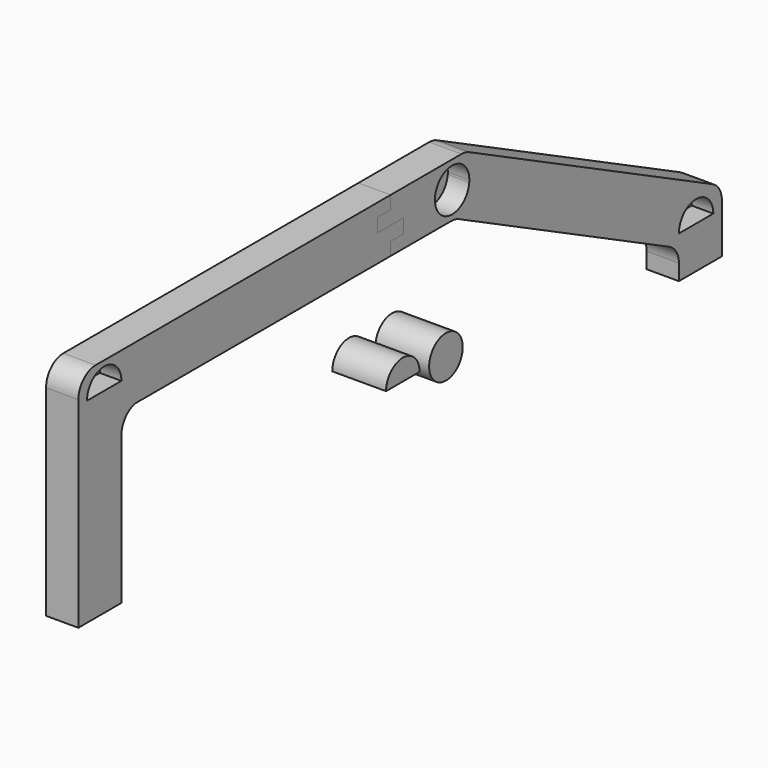
from build123d import *

# Parameters (mm, degrees)
F3_DEPTH  = 15
F4_DEPTH  = 25
F5_DEPTH  = 15
F6_DEPTH  = 25
F7_DEPTH  = 25
F8_R      = 9.75
F9_DEPTH  = 25
F10_DEPTH = 5
F11_DEPTH = 5
F12_DEPTH = 5


with BuildPart() as f3:
    # F2 (on Right) → F3 (new body)
    with BuildSketch(Plane.YZ):
        with BuildLine():
            Line((-64.0537443757, -47.7458898533), (-64.0537443757, -41.7458898533))
            Line((-64.0537443757, -41.7458898533), (-235.4606981414, -41.7458898533))
            ThreePointArc((-235.4606981414, -41.7458898533), (-242.5317659533, -44.6748220415), (-245.4606981414, -51.7458898533))
            Line((-245.4606981414, -51.7458898533), (-245.4606981414, -145.1103440631))
            Line((-245.4606981414, -145.1103440631), (-220.4606981414, -145.1103440631))
            Line((-220.4606981414, -145.1103440631), (-220.4606981414, -76.5684022923))
            ThreePointArc((-220.4606981414, -76.5684022923), (-218.1664426563, -70.1949023534), (-212.336397847, -66.7458898533))
            Line((-212.336397847, -66.7458898533), (-64.0537443757, -66.7458898533))
            Line((-64.0537443757, -66.7458898533), (-64.0537443757, -60.7458898533))
            Line((-64.0537443757, -60.7458898533), (-56.5537443757, -60.7458898533))
            Line((-56.5537443757, -60.7458898533), (-56.5537443757, -54.18692423))
            Line((-56.5537443757, -54.18692423), (-71.5537443757, -54.18692423))
            Line((-71.5537443757, -54.18692423), (-71.5537443757, -47.7458898533))
            Line((-71.5537443757, -47.7458898533), (-64.0537443757, -47.7458898533))
        make_face()
    extrude(amount=F3_DEPTH)

    # F1 (on Right) → F4 (cut)
    with BuildSketch(Plane.YZ):
        with BuildLine():
            Line((-230.4606981414, -54.2458898533), (-220.4606981414, -54.2458898533))
            ThreePointArc((-220.4606981414, -54.2458898533), (-230.4606981414, -44.2458898533), (-240.4606981414, -54.2458898533))
            Line((-240.4606981414, -54.2458898533), (-230.4606981414, -54.2458898533))
        make_face()
    extrude(amount=F4_DEPTH, mode=Mode.SUBTRACT)

    # F1 (on Right) → F10 (join)
    with BuildSketch(Plane.YZ):
        with BuildLine():
            Line((-230.4606981414, -54.2458898533), (-220.4606981414, -54.2458898533))
            ThreePointArc((-220.4606981414, -54.2458898533), (-230.4606981414, -44.2458898533), (-240.4606981414, -54.2458898533))
            Line((-240.4606981414, -54.2458898533), (-230.4606981414, -54.2458898533))
        make_face()
    extrude(amount=F10_DEPTH)


with BuildPart() as f5:
    # F2 (on Right) → F5 (new body)
    with BuildSketch(Plane.YZ):
        with BuildLine():
            Line((103.3974266851, -145.1103440631), (128.3974266851, -145.1103440631))
            Line((128.3974266851, -145.1103440631), (128.3974266851, -122.2802950504))
            ThreePointArc((128.3974266851, -122.2802950504), (126.9020431462, -117.0199244505), (122.8631269154, -113.3328081712))
            Line((122.8631269154, -113.3328081712), (-18.4597660903, -42.7984017651))
            ThreePointArc((-18.4597660903, -42.7984017651), (-20.6290450089, -42.0131372779), (-22.9205489159, -41.7458898533))
            Line((-22.9205489159, -41.7458898533), (-64.0537443757, -41.7458898533))
            Line((-64.0537443757, -41.7458898533), (-64.0537443757, -47.7458898533))
            Line((-64.0537443757, -47.7458898533), (-71.5537443757, -47.7458898533))
            Line((-71.5537443757, -47.7458898533), (-71.5537443757, -54.18692423))
            Line((-71.5537443757, -54.18692423), (-56.5537443757, -54.18692423))
            Line((-56.5537443757, -54.18692423), (-56.5537443757, -60.7458898533))
            Line((-56.5537443757, -60.7458898533), (-64.0537443757, -60.7458898533))
            Line((-64.0537443757, -60.7458898533), (-64.0537443757, -66.7458898533))
            Line((-64.0537443757, -66.7458898533), (-28.8176704198, -66.7458898533))
            ThreePointArc((-28.8176704198, -66.7458898533), (-26.5236421715, -67.0125741595), (-24.3519701895, -67.7984029742))
            Line((-24.3519701895, -67.7984029742), (97.8631269154, -128.7960880966))
            ThreePointArc((97.8631269154, -128.7960880966), (101.9020431462, -132.4832043759), (103.3974266851, -137.7435749758))
            Line((103.3974266851, -137.7435749758), (103.3974266851, -145.1103440631))
        make_face()
    extrude(amount=F5_DEPTH)

    # F1 (on Right) → F6 (cut)
    with BuildSketch(Plane.YZ):
        with BuildLine():
            Line((-28.3260242226, -54.2458898533), (-18.3260242226, -54.2458898533))
            ThreePointArc((-18.3260242226, -54.2458898533), (-28.3260242226, -44.2458898533), (-38.3260242226, -54.2458898533))
            Line((-38.3260242226, -54.2458898533), (-28.3260242226, -54.2458898533))
        make_face()
    extrude(amount=F6_DEPTH, mode=Mode.SUBTRACT)

    # F1 (on Right) → F7 (cut)
    with BuildSketch(Plane.YZ):
        with BuildLine():
            ThreePointArc((123.3974266851, -125.5894405546), (117.4455848239, -116.4454580698), (106.6749435485, -118.1861831311))
            ThreePointArc((106.6749435485, -118.1861831311), (104.2534442002, -121.5412824158), (103.3974266851, -125.5894405546))
            Line((103.3974266851, -125.5894405546), (113.3974266851, -125.5894405546))
            Line((113.3974266851, -125.5894405546), (123.3974266851, -125.5894405546))
        make_face()
        with BuildLine():
            ThreePointArc((-18.3751599266, -55.2359907384), (-18.3383157026, -54.741549535), (-18.3260242226, -54.2458898533))
            Line((-18.3260242226, -54.2458898533), (-28.3260242226, -54.2458898533))
            Line((-28.3260242226, -54.2458898533), (-38.3260242226, -54.2458898533))
            ThreePointArc((-38.3260242226, -54.2458898533), (-28.8216839042, -64.2335983733), (-18.3751599266, -55.2359907384))
        make_face()
    extrude(amount=F7_DEPTH, mode=Mode.SUBTRACT)

    # F1 (on Right) → F11 (join)
    with BuildSketch(Plane.YZ):
        with BuildLine():
            Line((-28.3260242226, -54.2458898533), (-18.3260242226, -54.2458898533))
            ThreePointArc((-18.3260242226, -54.2458898533), (-28.3260242226, -44.2458898533), (-38.3260242226, -54.2458898533))
            Line((-38.3260242226, -54.2458898533), (-28.3260242226, -54.2458898533))
        make_face()
        with BuildLine():
            ThreePointArc((123.3974266851, -125.5894405546), (117.4455848239, -116.4454580698), (106.6749435485, -118.1861831311))
            ThreePointArc((106.6749435485, -118.1861831311), (104.2534442002, -121.5412824158), (103.3974266851, -125.5894405546))
            Line((103.3974266851, -125.5894405546), (113.3974266851, -125.5894405546))
            Line((113.3974266851, -125.5894405546), (123.3974266851, -125.5894405546))
        make_face()
    extrude(amount=F11_DEPTH)

    # F1 (on Right) → F12 (join)
    with BuildSketch(Plane.YZ):
        with BuildLine():
            ThreePointArc((-18.3751599266, -55.2359907384), (-18.3383157026, -54.741549535), (-18.3260242226, -54.2458898533))
            Line((-18.3260242226, -54.2458898533), (-28.3260242226, -54.2458898533))
            Line((-28.3260242226, -54.2458898533), (-38.3260242226, -54.2458898533))
            ThreePointArc((-38.3260242226, -54.2458898533), (-28.8216839042, -64.2335983733), (-18.3751599266, -55.2359907384))
        make_face()
    extrude(amount=F12_DEPTH)


with BuildPart() as f9:
    # F8 (on Right) → F9 (new body)
    with BuildSketch(Plane.YZ):
        with Locations((-44.4301724343, -112.7188607796)):
            Circle(F8_R)
    extrude(amount=F9_DEPTH)


with BuildPart() as f9b:
    # F8 (on Right) → F9, piece 2 (new body)
    with BuildSketch(Plane.YZ):
        with BuildLine():
            Line((-69.4746359646, -112.642429769), (-59.7246359646, -112.642429769))
            ThreePointArc((-59.7246359646, -112.642429769), (-69.4746359646, -102.892429769), (-79.2246359646, -112.642429769))
            Line((-79.2246359646, -112.642429769), (-69.4746359646, -112.642429769))
        make_face()
    extrude(amount=F9_DEPTH)


solid = Compound([f3.part, f5.part, f9.part, f9b.part])
